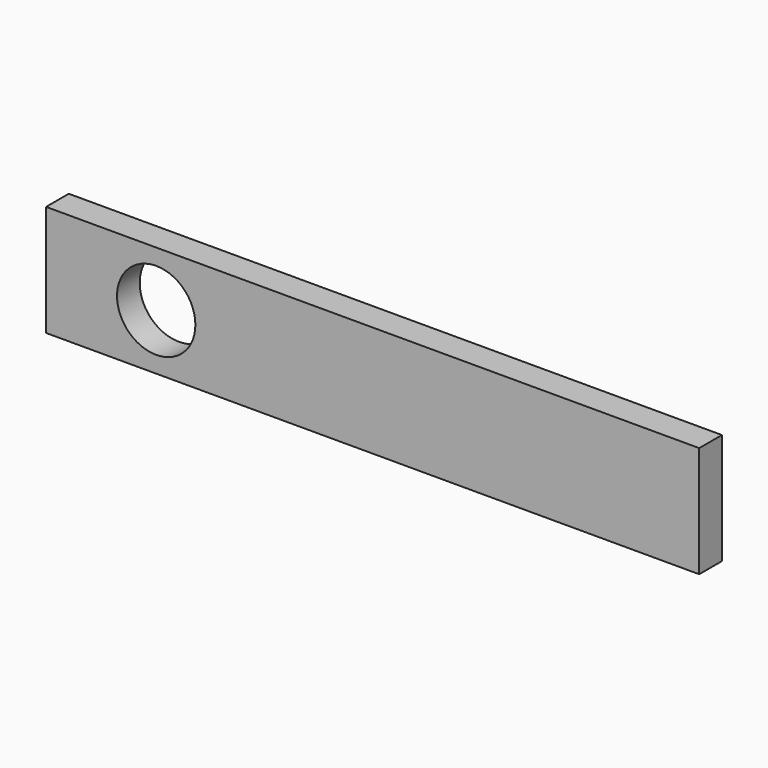
from build123d import *

# Parameters (mm, degrees)
F0_W     = 127
F0_H     = 21.59
F0_R     = 7.62
F1_DEPTH = 5.5170031264


# Not quite as in the source:
# - the program builds the solid bodies; features that only make, move or delete a surface that nothing else refers to are left out


with BuildPart() as f1:
    # F0 (on Front) → F1 (new body)
    with BuildSketch(Plane.XZ):
        with Locations((14.6961806784, 11.4298760891)):
            Rectangle(F0_W, F0_H)
        with Locations((-27.3933932185, 11.4667490125)):
            Circle(F0_R, mode=Mode.SUBTRACT)
    extrude(amount=F1_DEPTH)


solid = f1.part
